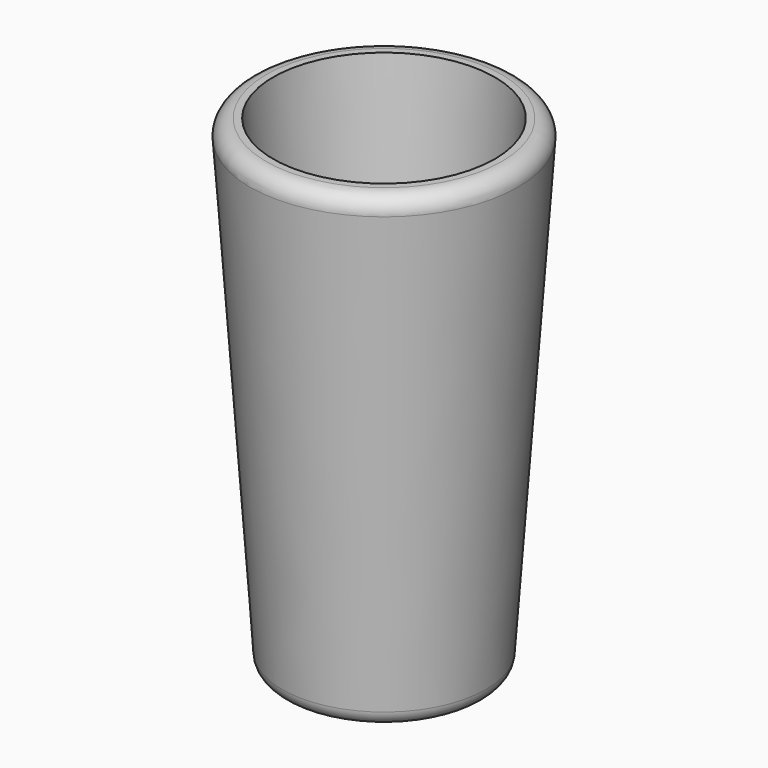
from build123d import *

# Parameters (mm, degrees)
F0_R = 31.75
F2_R = 42.4803799305
F4_T = -7.62
F5_R = 5.08
F6_R = 5.08
F7_R = 5.08


with BuildPart() as f3:
    # F0 (on Top) → F3 section 0
    with BuildSketch(Plane.XY):
        Circle(F0_R)
    # F2 (on offset) → F3 section 1
    with BuildSketch(Plane.XY.offset(152.4)):
        Circle(F2_R)
    loft()

    # F4
    f4_openings = [f3.faces().sort_by_distance(p)[0] for p in [
        (0, 0, 152.4),
    ]]
    offset(amount=F4_T, openings=f4_openings, kind=Kind.INTERSECTION)

    # F5
    f5_edges = [f3.edges().sort_by_distance(p)[0] for p in [
        (-42.48038, 0, 152.4),
    ]]
    fillet(f5_edges, radius=F5_R)

    # F6
    f6_edges = [f3.edges().sort_by_distance(p)[0] for p in [
        (-31.75, 0, 0),
    ]]
    fillet(f6_edges, radius=F6_R)

    # F7
    f7_edges = [f3.edges().sort_by_distance(p)[0] for p in [
        (-24.647654, 0, 7.62),
    ]]
    fillet(f7_edges, radius=F7_R)


solid = f3.part
